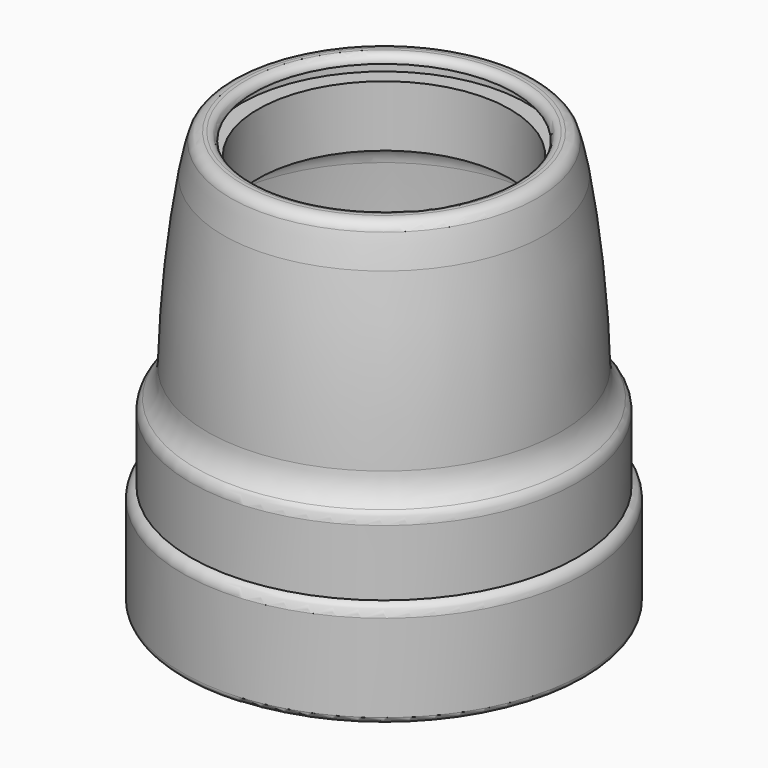
from build123d import *

# Parameters (mm, degrees)
F2_R = 1.49999


# Not quite as in the source:
# - a fillet or chamfer is up to 0.001 mm smaller than in the source, because OpenCascade refuses the exact size


with BuildPart() as f1:
    # F0 (on Front) → F1 (revolve)
    with BuildSketch(Plane.XZ):
        with BuildLine():
            Line((47.5, -7.8858422488), (47.5, -21.8858422488))
            Line((47.5, -21.8858422488), (48, -21.8858422488))
            Line((48, -21.8858422488), (48, -22.8858422488))
            Line((48, -22.8858422488), (46.5, -22.8858422488))
            Line((46.5, -22.8858422488), (46.5, -30.8858422488))
            Line((46.5, -30.8858422488), (49.5, -30.8858422488))
            Line((49.5, -30.8858422488), (49.5, -7.8858422488))
            ThreePointArc((49.5, -7.8858422488), (48.9494897428, -6.1537914412), (47.5, -5.0574151241))
            Line((47.5, -5.0574151241), (47.5, 11.1141577512))
            ThreePointArc((47.5, 11.1141577512), (47.1970669824, 12.6411468564), (46.3341521363, 13.9368482529))
            ThreePointArc((46.3341521363, 13.9368482529), (44.2221465916, 17.0682601408), (43.4222684299, 20.7596694596))
            ThreePointArc((43.4222684299, 20.7596694596), (42.1842659663, 41.4253133381), (39.4446819312, 61.9459411631))
            ThreePointArc((39.4446819312, 61.9459411631), (38.6802297275, 65.7174308689), (37.6848888881, 69.4346634937))
            ThreePointArc((37.6848888881, 69.4346634937), (36.6018643239, 70.9775375054), (34.8122661503, 71.5697712424))
            Line((34.8122661503, 71.5697712424), (34, 71.5697712424))
            ThreePointArc((34, 71.5697712424), (32.5857864376, 70.9839848048), (32, 69.5697712424))
            Line((32, 69.5697712424), (35, 69.5697712424))
            Line((35, 69.5697712424), (35, 66.3697712424))
            Line((35, 66.3697712424), (30.9395619044, 66.3697712424))
            Line((30.9395619044, 66.3697712424), (30.9395619044, 51.3697712424))
            Line((30.9395619044, 51.3697712424), (32.9395619044, 51.3697712424))
            Line((32.9395619044, 51.3697712424), (32.9395619044, 50.3697712424))
            ThreePointArc((32.9395619044, 50.3697712424), (37.6190355898, 48.5762120979), (39.9003508649, 44.1141577512))
            ThreePointArc((39.9003508649, 44.1141577512), (41.0998038622, 29.1354665936), (41.5, 14.1141577512))
            ThreePointArc((41.5, 14.1141577512), (41.7928932188, 13.40705097), (42.5, 13.1141577512))
            Line((42.5, 13.1141577512), (43.5, 13.1141577512))
            ThreePointArc((43.5, 13.1141577512), (44.9142135624, 12.5283713136), (45.5, 11.1141577512))
            Line((45.5, 11.1141577512), (45.5, -6.3858422488))
            ThreePointArc((45.5, -6.3858422488), (45.6464466094, -6.7393956394), (46, -6.8858422488))
            Line((46, -6.8858422488), (46.5, -6.8858422488))
            ThreePointArc((46.5, -6.8858422488), (47.2071067812, -7.1787354676), (47.5, -7.8858422488))
        make_face()
    revolve(axis=Axis((0, 0, 19.4899514318), (0, 0, 1)))

    # F2 (radius 1.5 in the source; OpenCascade refuses exactly that, so slightly less here)
    f2_edges = [f1.edges().sort_by_distance(p)[0] for p in [
        (-49.5, 0, -30.885842),
        (-46.5, 0, -30.885842),
    ]]
    fillet(f2_edges, radius=F2_R)


solid = f1.part
